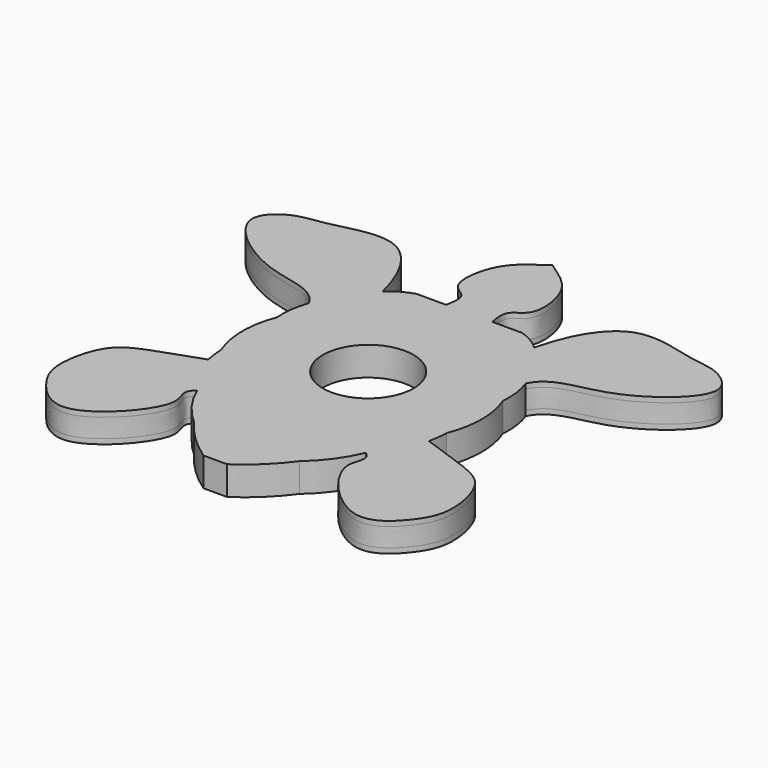
from build123d import *

# Parameters (mm, degrees)
F0_R     = 11
F0_R_2   = 9.525
F1_DEPTH = 4.56
F2_R     = 9.525
F2_R_2   = 11
F3_DEPTH = 1.22
F4_R     = 9.525
F4_R_2   = 11
F5_DEPTH = 1.22


with BuildPart() as f1:
    # F0 (on Top) → F1 (new body)
    with BuildSketch(Plane.XY):
        with BuildLine():
            Line((5.625097611, 30.6178405881), (0, 30.6178405881))
            Line((0, 30.6178405881), (-5.625097611, 30.6178405881))
            Line((-5.625097611, 30.6178405881), (-12.7985710278, 30.6178405881))
            ThreePointArc((-12.7985710278, 30.6178405881), (-15.7869475666, 29.3230184651), (-18.3888467007, 27.364171977))
            ThreePointArc((-18.3888467007, 27.364171977), (-20.4594688448, 24.8503138656), (-21.8835807745, 21.9213441014))
            ThreePointArc((-21.8835807745, 21.9213441014), (-24.482449048, 18.6236111214), (-26.320533588, 14.8486138585))
            ThreePointArc((-26.320533588, 14.8486138585), (-27.3137379545, 10.7690668007), (-27.4166208475, 6.5716182636))
            ThreePointArc((-27.4166208475, 6.5716182636), (-28.9941311969, -1.9294271862), (-27.3426556245, -10.4164137584))
            ThreePointArc((-27.3426556245, -10.4164137584), (-27.160991282, -12.7450107701), (-26.7452726242, -15.0433893234))
            ThreePointArc((-26.7452726242, -15.0433893234), (-24.3962536961, -21.0937392774), (-20.4578898847, -26.2526068836))
            ThreePointArc((-20.4578898847, -26.2526068836), (-17.2427631702, -31.9653205751), (-12.7985710278, -36.7841683328))
            ThreePointArc((-12.7985710278, -36.7841683328), (-8.2428664491, -42.0110098773), (-2.8414558619, -46.3583171368))
            Line((-2.8414558619, -46.3583171368), (0, -46.3583171368))
            Line((0, -46.3583171368), (2.8414558619, -46.3583171368))
            ThreePointArc((2.8414558619, -46.3583171368), (8.2428664491, -42.0110098773), (12.7985710278, -36.7841683328))
            ThreePointArc((12.7985710278, -36.7841683328), (17.2427631702, -31.9653205751), (20.4578898847, -26.2526068836))
            ThreePointArc((20.4578898847, -26.2526068836), (24.3962536961, -21.0937392774), (26.7452726242, -15.0433893234))
            ThreePointArc((26.7452726242, -15.0433893234), (27.160991282, -12.7450107701), (27.3426556245, -10.4164137584))
            ThreePointArc((27.3426556245, -10.4164137584), (28.9941311969, -1.9294271862), (27.4166208475, 6.5716182636))
            ThreePointArc((27.4166208475, 6.5716182636), (27.3137379545, 10.7690668007), (26.320533588, 14.8486138585))
            ThreePointArc((26.320533588, 14.8486138585), (24.482449048, 18.6236111214), (21.8835807745, 21.9213441014))
            ThreePointArc((21.8835807745, 21.9213441014), (20.4594688448, 24.8503138656), (18.3888467007, 27.364171977))
            ThreePointArc((18.3888467007, 27.364171977), (15.7869475666, 29.3230184651), (12.7985710278, 30.6178405881))
            Line((12.7985710278, 30.6178405881), (5.625097611, 30.6178405881))
        make_face()
        Circle(F0_R, mode=Mode.SUBTRACT)
        with BuildLine():
            Line((-5.625097611, 30.6178405881), (0, 30.6178405881))
            Line((0, 30.6178405881), (5.625097611, 30.6178405881))
            add(Edge.make_bspline(
                [(5.625097611, 30.6178405881), (5.3087040961, 32.1895229994), (4.568154115, 35.9491431064), (10.5811975265, 37.4321097713), (8.8632431136, 49.383446037), (3.2061824976, 53.6620796768), (0.9419427303, 55.2415959276), (0, 55.8932051063)],
                knots=[0, 0, 0, 0, 0.1784283658, 0.3531222021, 0.6190719873, 0.8402365752, 1, 1, 1, 1], degree=3))
            add(Edge.make_bspline(
                [(-5.625097611, 30.6178405881), (-5.3087040961, 32.1895229994), (-4.568154115, 35.9491431064), (-10.5811975265, 37.4321097713), (-8.8632431136, 49.383446037), (-3.2061824976, 53.6620796768), (-0.9419427303, 55.2415959276), (0, 55.8932051063)],
                knots=[0, 0, 0, 0, 0.1784283658, 0.3531222021, 0.6190719873, 0.8402365752, 1, 1, 1, 1], degree=3))
        make_face()
        with BuildLine():
            ThreePointArc((-21.8835807745, 21.9213441014), (-20.4594688448, 24.8503138656), (-18.3888467007, 27.364171977))
            add(Edge.make_bspline(
                [(-18.3888467007, 27.364171977), (-20.2840508895, 35.2449831328), (-27.1514149225, 48.0960335812), (-44.0946491651, 41.9492612732), (-51.1984685962, 42.077927417), (-60.7459841372, 34.3488029627), (-41.5970901495, 18.9610148145), (-28.8989599794, 20.0606454164), (-26.320533588, 14.8486138585)],
                knots=[0, 0, 0, 0, 0.1995819174, 0.371038677, 0.4943928252, 0.6184057886, 0.8173226516, 1, 1, 1, 1], degree=3))
            ThreePointArc((-26.320533588, 14.8486138585), (-24.482449048, 18.6236111214), (-21.8835807745, 21.9213441014))
        make_face()
        with Locations((-34.4810523093, 31.9225937128)):
            Circle(F0_R_2, mode=Mode.SUBTRACT)
        with BuildLine():
            add(Edge.make_bspline(
                [(18.3888467007, 27.364171977), (20.2840508895, 35.2449831328), (27.1514149225, 48.0960335812), (44.0946491651, 41.9492612732), (51.1984685962, 42.077927417), (60.7459841372, 34.3488029627), (41.5970901495, 18.9610148145), (28.8989599794, 20.0606454164), (26.320533588, 14.8486138585)],
                knots=[0, 0, 0, 0, 0.1995819174, 0.371038677, 0.4943928252, 0.6184057886, 0.8173226516, 1, 1, 1, 1], degree=3))
            ThreePointArc((18.3888467007, 27.364171977), (20.4594688448, 24.8503138656), (21.8835807745, 21.9213441014))
            ThreePointArc((21.8835807745, 21.9213441014), (24.482449048, 18.6236111214), (26.320533588, 14.8486138585))
        make_face()
        with Locations((34.4810523093, 31.9225937128)):
            Circle(F0_R_2, mode=Mode.SUBTRACT)
        with BuildLine():
            ThreePointArc((-20.4578898847, -26.2526068836), (-24.3962536961, -21.0937392774), (-26.7452726242, -15.0433893234))
            add(Edge.make_bspline(
                [(-26.7452726242, -15.0433893234), (-31.393476313, -16.8312141012), (-39.3754850186, -19.1220217061), (-45.7883974033, -23.0677833544), (-48.5542379231, -34.7892824207), (-45.1601303547, -42.145527965), (-34.6295665467, -52.3597202212), (-16.9151388877, -32.4850856335), (-23.0679627748, -28.326411455), (-20.4578898847, -26.2526068836)],
                knots=[0, 0, 0, 0, 0.1609366377, 0.2773333927, 0.4214369084, 0.5475288587, 0.6931611492, 0.8900357357, 1, 1, 1, 1], degree=3))
        make_face()
        with Locations((-34.4810523093, -31.9225937128)):
            Circle(F0_R_2, mode=Mode.SUBTRACT)
        with BuildLine():
            add(Edge.make_bspline(
                [(26.7452726242, -15.0433893234), (31.393476313, -16.8312141012), (39.3754850186, -19.1220217061), (45.7883974033, -23.0677833544), (48.5542379231, -34.7892824207), (45.1601303547, -42.145527965), (34.6295665467, -52.3597202212), (16.9151388877, -32.4850856335), (23.0679627748, -28.326411455), (20.4578898847, -26.2526068836)],
                knots=[0, 0, 0, 0, 0.1609366377, 0.2773333927, 0.4214369084, 0.5475288587, 0.6931611492, 0.8900357357, 1, 1, 1, 1], degree=3))
            ThreePointArc((26.7452726242, -15.0433893234), (24.3962536961, -21.0937392774), (20.4578898847, -26.2526068836))
        make_face()
        with Locations((34.4810523093, -31.9225937128)):
            Circle(F0_R_2, mode=Mode.SUBTRACT)
    extrude(amount=F1_DEPTH)

    # F2 (on face) → F3 (join)
    with BuildSketch(Plane(origin=(0, 0, 0), x_dir=(1, 0, 0), z_dir=(0, 0, -1))):
        with BuildLine():
            add(Edge.make_bspline(
                [(18.3888467007, -27.364171977), (20.2840508895, -35.2449831328), (27.1514149225, -48.0960335812), (44.0946491651, -41.9492612732), (51.1984685962, -42.077927417), (60.7459841372, -34.3488029627), (41.5970901495, -18.9610148145), (28.8989599794, -20.0606454164), (26.320533588, -14.8486138585)],
                knots=[0, 0, 0, 0, 0.1995819174, 0.371038677, 0.4943928252, 0.6184057886, 0.8173226516, 1, 1, 1, 1], degree=3))
            ThreePointArc((26.320533588, -14.8486138585), (27.3137379545, -10.7690668007), (27.4166208475, -6.5716182636))
            ThreePointArc((27.4166208475, -6.5716182636), (28.9941311969, 1.9294271862), (27.3426556245, 10.4164137584))
            ThreePointArc((27.3426556245, 10.4164137584), (27.160991282, 12.7450107701), (26.7452726242, 15.0433893234))
            add(Edge.make_bspline(
                [(26.7452726242, 15.0433893234), (31.393476313, 16.8312141012), (39.3754850186, 19.1220217061), (45.7883974033, 23.0677833544), (48.5542379231, 34.7892824207), (45.1601303547, 42.145527965), (34.6295665467, 52.3597202212), (16.9151388877, 32.4850856335), (23.0679627748, 28.326411455), (20.4578898847, 26.2526068836)],
                knots=[0, 0, 0, 0, 0.1609366377, 0.2773333927, 0.4214369084, 0.5475288587, 0.6931611492, 0.8900357357, 1, 1, 1, 1], degree=3))
            ThreePointArc((20.4578898847, 26.2526068836), (17.2427631702, 31.9653205751), (12.7985710278, 36.7841683328))
            ThreePointArc((12.7985710278, 36.7841683328), (8.2428664491, 42.0110098773), (2.8414558619, 46.3583171368))
            Line((2.8414558619, 46.3583171368), (-2.8414558619, 46.3583171368))
            ThreePointArc((-2.8414558619, 46.3583171368), (-8.2428664491, 42.0110098773), (-12.7985710278, 36.7841683328))
            ThreePointArc((-12.7985710278, 36.7841683328), (-17.2427631702, 31.9653205751), (-20.4578898847, 26.2526068836))
            add(Edge.make_bspline(
                [(-26.7452726242, 15.0433893234), (-31.393476313, 16.8312141012), (-39.3754850186, 19.1220217061), (-45.7883974033, 23.0677833544), (-48.5542379231, 34.7892824207), (-45.1601303547, 42.145527965), (-34.6295665467, 52.3597202212), (-16.9151388877, 32.4850856335), (-23.0679627748, 28.326411455), (-20.4578898847, 26.2526068836)],
                knots=[0, 0, 0, 0, 0.1609366377, 0.2773333927, 0.4214369084, 0.5475288587, 0.6931611492, 0.8900357357, 1, 1, 1, 1], degree=3))
            ThreePointArc((-26.7452726242, 15.0433893234), (-27.160991282, 12.7450107701), (-27.3426556245, 10.4164137584))
            ThreePointArc((-27.3426556245, 10.4164137584), (-28.9941311969, 1.9294271862), (-27.4166208475, -6.5716182636))
            ThreePointArc((-27.4166208475, -6.5716182636), (-27.3137379545, -10.7690668007), (-26.320533588, -14.8486138585))
            add(Edge.make_bspline(
                [(-18.3888467007, -27.364171977), (-20.2840508895, -35.2449831328), (-27.1514149225, -48.0960335812), (-44.0946491651, -41.9492612732), (-51.1984685962, -42.077927417), (-60.7459841372, -34.3488029627), (-41.5970901495, -18.9610148145), (-28.8989599794, -20.0606454164), (-26.320533588, -14.8486138585)],
                knots=[0, 0, 0, 0, 0.1995819174, 0.371038677, 0.4943928252, 0.6184057886, 0.8173226516, 1, 1, 1, 1], degree=3))
            ThreePointArc((-18.3888467007, -27.364171977), (-15.7869475666, -29.3230184651), (-12.7985710278, -30.6178405881))
            Line((-12.7985710278, -30.6178405881), (-5.625097611, -30.6178405881))
            add(Edge.make_bspline(
                [(-5.625097611, -30.6178405881), (-5.3087040961, -32.1895229994), (-4.568154115, -35.9491431064), (-10.5811975265, -37.4321097713), (-8.8632431136, -49.383446037), (-3.2061824976, -53.6620796768), (-0.9419427303, -55.2415959276), (0, -55.8932051063)],
                knots=[0, 0, 0, 0, 0.1784283658, 0.3531222021, 0.6190719873, 0.8402365752, 1, 1, 1, 1], degree=3))
            add(Edge.make_bspline(
                [(5.625097611, -30.6178405881), (5.3087040961, -32.1895229994), (4.568154115, -35.9491431064), (10.5811975265, -37.4321097713), (8.8632431136, -49.383446037), (3.2061824976, -53.6620796768), (0.9419427303, -55.2415959276), (0, -55.8932051063)],
                knots=[0, 0, 0, 0, 0.1784283658, 0.3531222021, 0.6190719873, 0.8402365752, 1, 1, 1, 1], degree=3))
            Line((5.625097611, -30.6178405881), (12.7985710278, -30.6178405881))
            ThreePointArc((12.7985710278, -30.6178405881), (15.7869475666, -29.3230184651), (18.3888467007, -27.364171977))
        make_face()
        with Locations((-34.4810523093, -31.9225937128)):
            Circle(F2_R, mode=Mode.SUBTRACT)
        with Locations((34.4810523093, -31.9225937128)):
            Circle(F2_R, mode=Mode.SUBTRACT)
        Circle(F2_R_2, mode=Mode.SUBTRACT)
        with Locations((-34.4810523093, 31.9225937128)):
            Circle(F2_R, mode=Mode.SUBTRACT)
        with Locations((34.4810523093, 31.9225937128)):
            Circle(F2_R, mode=Mode.SUBTRACT)
        with Locations((-34.4810523093, 31.9225937128)):
            Circle(F2_R)
        with Locations((34.4810523093, 31.9225937128)):
            Circle(F2_R)
        with Locations((-34.4810523093, -31.9225937128)):
            Circle(F2_R)
        with Locations((34.4810523093, -31.9225937128)):
            Circle(F2_R)
    extrude(amount=F3_DEPTH)

    # F4 (on face) → F5 (join)
    with BuildSketch(Plane.XY.offset(4.56)):
        with BuildLine():
            ThreePointArc((27.3426556245, -10.4164137584), (28.9941311969, -1.9294271862), (27.4166208475, 6.5716182636))
            ThreePointArc((27.4166208475, 6.5716182636), (27.3137379545, 10.7690668007), (26.320533588, 14.8486138585))
            add(Edge.make_bspline(
                [(18.3888467007, 27.364171977), (20.2840508895, 35.2449831328), (27.1514149225, 48.0960335812), (44.0946491651, 41.9492612732), (51.1984685962, 42.077927417), (60.7459841372, 34.3488029627), (41.5970901495, 18.9610148145), (28.8989599794, 20.0606454164), (26.320533588, 14.8486138585)],
                knots=[0, 0, 0, 0, 0.1995819174, 0.371038677, 0.4943928252, 0.6184057886, 0.8173226516, 1, 1, 1, 1], degree=3))
            ThreePointArc((18.3888467007, 27.364171977), (15.7869475666, 29.3230184651), (12.7985710278, 30.6178405881))
            Line((12.7985710278, 30.6178405881), (5.625097611, 30.6178405881))
            add(Edge.make_bspline(
                [(5.625097611, 30.6178405881), (5.3087040961, 32.1895229994), (4.568154115, 35.9491431064), (10.5811975265, 37.4321097713), (8.8632431136, 49.383446037), (3.2061824976, 53.6620796768), (0.9419427303, 55.2415959276), (0, 55.8932051063)],
                knots=[0, 0, 0, 0, 0.1784283658, 0.3531222021, 0.6190719873, 0.8402365752, 1, 1, 1, 1], degree=3))
            add(Edge.make_bspline(
                [(-5.625097611, 30.6178405881), (-5.3087040961, 32.1895229994), (-4.568154115, 35.9491431064), (-10.5811975265, 37.4321097713), (-8.8632431136, 49.383446037), (-3.2061824976, 53.6620796768), (-0.9419427303, 55.2415959276), (0, 55.8932051063)],
                knots=[0, 0, 0, 0, 0.1784283658, 0.3531222021, 0.6190719873, 0.8402365752, 1, 1, 1, 1], degree=3))
            Line((-5.625097611, 30.6178405881), (-12.7985710278, 30.6178405881))
            ThreePointArc((-12.7985710278, 30.6178405881), (-15.7869475666, 29.3230184651), (-18.3888467007, 27.364171977))
            add(Edge.make_bspline(
                [(-18.3888467007, 27.364171977), (-20.2840508895, 35.2449831328), (-27.1514149225, 48.0960335812), (-44.0946491651, 41.9492612732), (-51.1984685962, 42.077927417), (-60.7459841372, 34.3488029627), (-41.5970901495, 18.9610148145), (-28.8989599794, 20.0606454164), (-26.320533588, 14.8486138585)],
                knots=[0, 0, 0, 0, 0.1995819174, 0.371038677, 0.4943928252, 0.6184057886, 0.8173226516, 1, 1, 1, 1], degree=3))
            ThreePointArc((-26.320533588, 14.8486138585), (-27.3137379545, 10.7690668007), (-27.4166208475, 6.5716182636))
            ThreePointArc((-27.4166208475, 6.5716182636), (-28.9941311969, -1.9294271862), (-27.3426556245, -10.4164137584))
            ThreePointArc((-27.3426556245, -10.4164137584), (-27.160991282, -12.7450107701), (-26.7452726242, -15.0433893234))
            add(Edge.make_bspline(
                [(-26.7452726242, -15.0433893234), (-31.393476313, -16.8312141012), (-39.3754850186, -19.1220217061), (-45.7883974033, -23.0677833544), (-48.5542379231, -34.7892824207), (-45.1601303547, -42.145527965), (-34.6295665467, -52.3597202212), (-16.9151388877, -32.4850856335), (-23.0679627748, -28.326411455), (-20.4578898847, -26.2526068836)],
                knots=[0, 0, 0, 0, 0.1609366377, 0.2773333927, 0.4214369084, 0.5475288587, 0.6931611492, 0.8900357357, 1, 1, 1, 1], degree=3))
            ThreePointArc((-20.4578898847, -26.2526068836), (-17.2427631702, -31.9653205751), (-12.7985710278, -36.7841683328))
            ThreePointArc((-12.7985710278, -36.7841683328), (-8.2428664491, -42.0110098773), (-2.8414558619, -46.3583171368))
            Line((-2.8414558619, -46.3583171368), (2.8414558619, -46.3583171368))
            ThreePointArc((2.8414558619, -46.3583171368), (8.2428664491, -42.0110098773), (12.7985710278, -36.7841683328))
            ThreePointArc((12.7985710278, -36.7841683328), (17.2427631702, -31.9653205751), (20.4578898847, -26.2526068836))
            add(Edge.make_bspline(
                [(26.7452726242, -15.0433893234), (31.393476313, -16.8312141012), (39.3754850186, -19.1220217061), (45.7883974033, -23.0677833544), (48.5542379231, -34.7892824207), (45.1601303547, -42.145527965), (34.6295665467, -52.3597202212), (16.9151388877, -32.4850856335), (23.0679627748, -28.326411455), (20.4578898847, -26.2526068836)],
                knots=[0, 0, 0, 0, 0.1609366377, 0.2773333927, 0.4214369084, 0.5475288587, 0.6931611492, 0.8900357357, 1, 1, 1, 1], degree=3))
            ThreePointArc((26.7452726242, -15.0433893234), (27.160991282, -12.7450107701), (27.3426556245, -10.4164137584))
        make_face()
        with Locations((-34.4810523093, -31.9225937128)):
            Circle(F4_R, mode=Mode.SUBTRACT)
        Circle(F4_R_2, mode=Mode.SUBTRACT)
        with Locations((34.4810523093, -31.9225937128)):
            Circle(F4_R, mode=Mode.SUBTRACT)
        with Locations((-34.4810523093, 31.9225937128)):
            Circle(F4_R, mode=Mode.SUBTRACT)
        with Locations((34.4810523093, 31.9225937128)):
            Circle(F4_R, mode=Mode.SUBTRACT)
        with Locations((-34.4810523093, 31.9225937128)):
            Circle(F4_R)
        with Locations((34.4810523093, 31.9225937128)):
            Circle(F4_R)
        with Locations((-34.4810523093, -31.9225937128)):
            Circle(F4_R)
        with Locations((34.4810523093, -31.9225937128)):
            Circle(F4_R)
    extrude(amount=F5_DEPTH)


solid = f1.part
